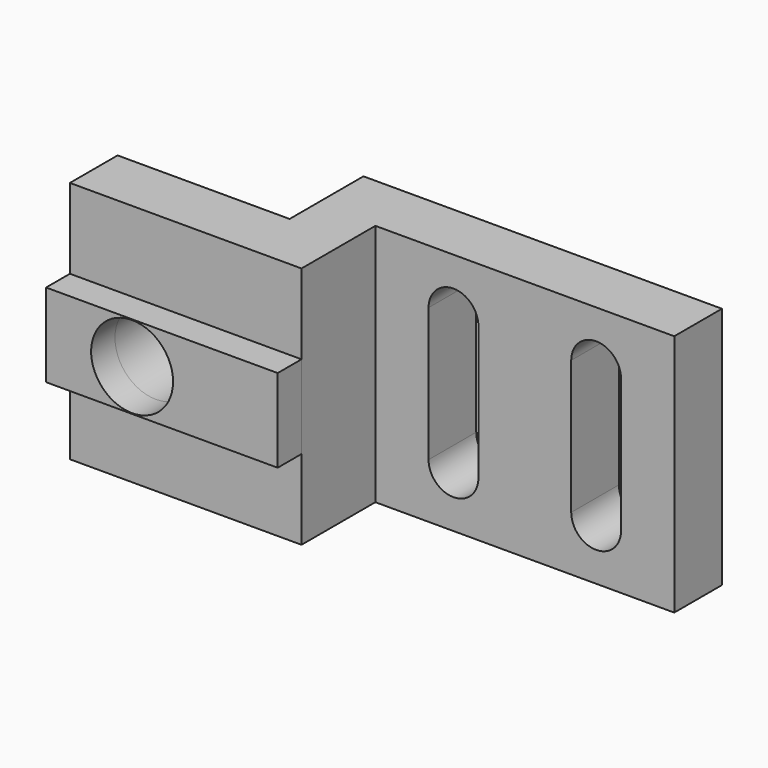
from build123d import *
from build123d import SkipClean  # not in build123d's __all__

# Parameters (mm, degrees)
F1_DEPTH = 8.167
F2_R     = 2.75
F3_DEPTH = 4.001
F5_DEPTH = 4.001
F6_W     = 15.549
F6_H     = 5.596
F6_R     = 2.75
F7_DEPTH = 2


with BuildPart() as f1:
    # F0 (on Top) → F1 (new body, symmetric)
    with BuildSketch(Plane.XY):
        Polygon((0, 4), (0, 0), (15.549, 0), (15.549, 6.1976), (35.615, 6.1976), (35.615, 10.1976), (11.549, 10.1976), (11.549, 4), align=None)
    extrude(amount=F1_DEPTH, both=True)

    # F2 (on face) → F3 (cut, through all)
    with BuildSketch(Plane(origin=(0, 4, 0), x_dir=(-1, 0, 0), z_dir=(0, 1, 0))):
        with Locations((-5.7745, 0)):
            Circle(F2_R)
    extrude(amount=-F3_DEPTH, mode=Mode.SUBTRACT)

    # F4 (on face) → F5 (cut, through all)
    with BuildSketch(Plane.XZ.offset(-6.1976)):
        with BuildLine():
            ThreePointArc((22.4665, 4.4946), (20.7941, 6.167), (19.1217, 4.4946))
            Line((19.1217, 4.4946), (19.1217, -4.4946))
            ThreePointArc((19.1217, -4.4946), (20.7941, -6.167), (22.4665, -4.4946))
            Line((22.4665, -4.4946), (22.4665, 4.4946))
        make_face()
        with BuildLine():
            ThreePointArc((32.0423, 4.4946), (30.3699, 6.167), (28.6975, 4.4946))
            Line((28.6975, 4.4946), (28.6975, -4.4946))
            ThreePointArc((28.6975, -4.4946), (30.3699, -6.167), (32.0423, -4.4946))
            Line((32.0423, -4.4946), (32.0423, 4.4946))
        make_face()
    extrude(amount=-F5_DEPTH, mode=Mode.SUBTRACT)

    # F6 (on face) → F7 (join)
    with BuildSketch(Plane.XZ):
        with Locations((7.7745, 0)):
            Rectangle(F6_W, F6_H)
        with Locations((5.7745, 0)):
            Circle(F6_R, mode=Mode.SUBTRACT)
    with SkipClean():  # cleaning this boolean's faces spoils the solid; the shape is the same uncleaned
        extrude(amount=F7_DEPTH)


solid = f1.part
